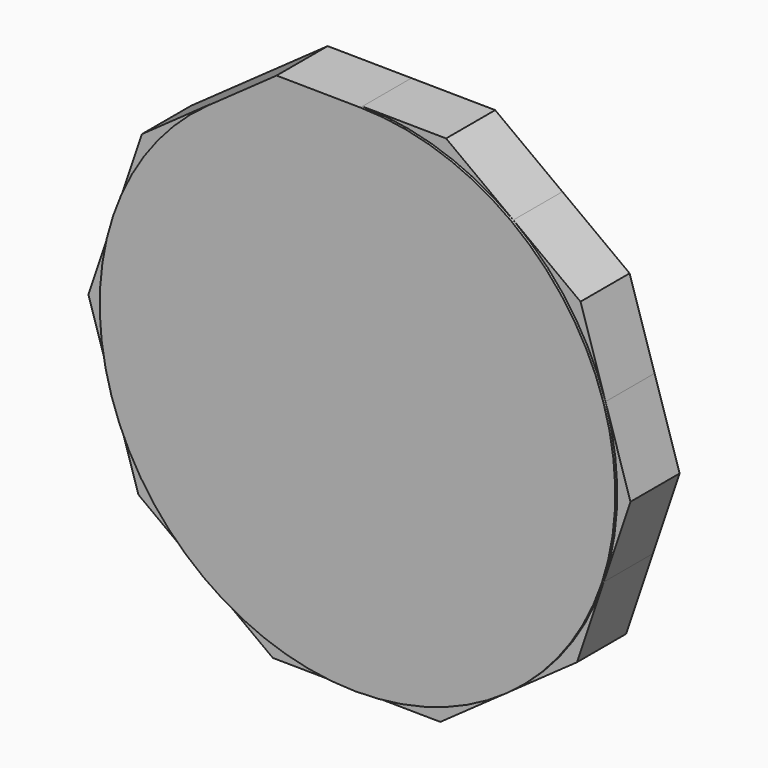
from build123d import *

# Parameters (mm, degrees)
F1_DEPTH = 1
F2_DEPTH = 25


with BuildPart() as f1:
    # F0 (on Front) → F1 (new body)
    with BuildSketch(Plane.XZ):
        with BuildLine():
            ThreePointArc((99.4907408065, -33.5647507629), (103.6135314153, -17.0069429252), (105, 0))
            ThreePointArc((105, 0), (103.7977584549, 15.8437792124), (100.2185649575, 31.3247384325))
            ThreePointArc((100.2185649575, 31.3247384325), (85.6336425012, 60.7608366629), (62.6663022671, 84.2492407097))
            ThreePointArc((62.6663022671, 84.2492407097), (33.5647485771, 99.4907415439), (1.1776435614, 104.9933957716))
            ThreePointArc((1.1776435614, 104.9933957716), (-31.3247392722, 100.218564695), (-60.7608381292, 85.6336414608))
            ThreePointArc((-60.7608381292, 85.6336414608), (-84.2492404255, 62.6663026493), (-99.4907409959, 33.5647502014))
            ThreePointArc((-99.4907409959, 33.5647502014), (-104.9933957718, 1.1776435403), (-100.2185647541, -31.3247390832))
            ThreePointArc((-100.2185647541, -31.3247390832), (-85.6336424849, -60.7608366859), (-62.6663027691, -84.2492403363))
            ThreePointArc((-62.6663027691, -84.2492403363), (-33.5647485613, -99.4907415492), (-1.1776429024, -104.9933957789))
            ThreePointArc((-1.1776429024, -104.9933957789), (31.3247396024, -100.2185645918), (60.7608381561, -85.6336414417))
            ThreePointArc((60.7608381561, -85.6336414417), (84.2492402585, -62.6663028738), (99.4907408065, -33.5647507629))
        make_face()
        with BuildLine():
            ThreePointArc((-60.7608381292, 85.6336414608), (-31.3247392722, 100.218564695), (1.1776435614, 104.9933957716))
            Line((1.1776435614, 104.9933957716), (-32.9367799888, 105.3760349567))
            Line((-32.9367799888, 105.3760349567), (-60.7608381292, 85.6336414608))
        make_face()
    extrude(amount=F1_DEPTH)

    # F0 (on Front) + F1_face (on face) → F2 (join)
    with BuildSketch(Plane.XZ):
        with BuildLine():
            ThreePointArc((99.4907408065, -33.5647507629), (103.6135314153, -17.0069429252), (105, 0))
            ThreePointArc((105, 0), (103.7977584549, 15.8437792124), (100.2185649575, 31.3247384325))
            ThreePointArc((100.2185649575, 31.3247384325), (85.6336425012, 60.7608366629), (62.6663022671, 84.2492407097))
            ThreePointArc((62.6663022671, 84.2492407097), (33.5647485771, 99.4907415439), (1.1776435614, 104.9933957716))
            ThreePointArc((1.1776435614, 104.9933957716), (-31.3247392722, 100.218564695), (-60.7608381292, 85.6336414608))
            ThreePointArc((-60.7608381292, 85.6336414608), (-84.2492404255, 62.6663026493), (-99.4907409959, 33.5647502014))
            ThreePointArc((-99.4907409959, 33.5647502014), (-104.9933957718, 1.1776435403), (-100.2185647541, -31.3247390832))
            ThreePointArc((-100.2185647541, -31.3247390832), (-85.6336424849, -60.7608366859), (-62.6663027691, -84.2492403363))
            ThreePointArc((-62.6663027691, -84.2492403363), (-33.5647485613, -99.4907415492), (-1.1776429024, -104.9933957789))
            ThreePointArc((-1.1776429024, -104.9933957789), (31.3247396024, -100.2185645918), (60.7608381561, -85.6336414417))
            ThreePointArc((60.7608381561, -85.6336414417), (84.2492402585, -62.6663028738), (99.4907408065, -33.5647507629))
        make_face()
        with BuildLine():
            ThreePointArc((100.2185649575, 31.3247384325), (103.7977584549, 15.8437792124), (105, 0))
            ThreePointArc((105, 0), (103.6135314153, -17.0069429252), (99.4907408065, -33.5647507629))
            Line((99.4907408065, -33.5647507629), (110.3965894634, -1.2382463674))
            Line((110.3965894634, -1.2382463674), (100.2185649575, 31.3247384325))
        make_face()
        with BuildLine():
            ThreePointArc((62.6663022671, 84.2492407097), (85.6336425012, 60.7608366629), (100.2185649575, 31.3247384325))
            Line((100.2185649575, 31.3247384325), (90.0405399504, 63.8877248356))
            Line((90.0405399504, 63.8877248356), (62.6663022671, 84.2492407097))
        make_face()
        with BuildLine():
            Line((88.5848940435, -65.8912495444), (99.4907408065, -33.5647507629))
            ThreePointArc((99.4907408065, -33.5647507629), (84.2492402585, -62.6663028738), (60.7608381561, -85.6336414417))
            Line((60.7608381561, -85.6336414417), (88.5848940435, -65.8912495444))
        make_face()
        with BuildLine():
            ThreePointArc((1.1776435614, 104.9933957716), (33.5647485771, 99.4907415439), (62.6663022671, 84.2492407097))
            Line((62.6663022671, 84.2492407097), (35.2920645417, 104.6107566152))
            Line((35.2920645417, 104.6107566152), (1.1776435614, 104.9933957716))
        make_face()
        with BuildLine():
            Line((32.9367799888, -105.3760349567), (60.7608381561, -85.6336414417))
            ThreePointArc((60.7608381561, -85.6336414417), (31.3247396024, -100.2185645918), (-1.1776429024, -104.9933957789))
            Line((-1.1776429024, -104.9933957789), (32.9367799888, -105.3760349567))
        make_face()
        with BuildLine():
            ThreePointArc((-60.7608381292, 85.6336414608), (-31.3247392722, 100.218564695), (1.1776435614, 104.9933957716))
            Line((1.1776435614, 104.9933957716), (-32.9367799888, 105.3760349567))
            Line((-32.9367799888, 105.3760349567), (-60.7608381292, 85.6336414608))
        make_face()
        with BuildLine():
            Line((-35.2920645417, -104.6107566152), (-1.1776429024, -104.9933957789))
            ThreePointArc((-1.1776429024, -104.9933957789), (-33.5647485613, -99.4907415492), (-62.6663027691, -84.2492403363))
            Line((-62.6663027691, -84.2492403363), (-35.2920645417, -104.6107566152))
        make_face()
        with BuildLine():
            ThreePointArc((-99.4907409959, 33.5647502014), (-84.2492404255, 62.6663026493), (-60.7608381292, 85.6336414608))
            Line((-60.7608381292, 85.6336414608), (-88.5848940435, 65.8912495444))
            Line((-88.5848940435, 65.8912495444), (-99.4907409959, 33.5647502014))
        make_face()
        with BuildLine():
            Line((-90.0405399504, -63.8877248356), (-62.6663027691, -84.2492403363))
            ThreePointArc((-62.6663027691, -84.2492403363), (-85.6336424849, -60.7608366859), (-100.2185647541, -31.3247390832))
            Line((-100.2185647541, -31.3247390832), (-90.0405399504, -63.8877248356))
        make_face()
        with BuildLine():
            ThreePointArc((-100.2185647541, -31.3247390832), (-104.9933957718, 1.1776435403), (-99.4907409959, 33.5647502014))
            Line((-99.4907409959, 33.5647502014), (-110.3965894634, 1.2382463674))
            Line((-110.3965894634, 1.2382463674), (-100.2185647541, -31.3247390832))
        make_face()
    with BuildSketch(Plane(origin=(-0.1080602071, -1, 0.3457215964), x_dir=(1, 0, 0), z_dir=(0, -1, 0))):
        with BuildLine():
            Line((1.2857037684, 104.6476741752), (-32.8287197817, 105.0303133603))
            Line((-32.8287197817, 105.0303133603), (-60.6527779221, 85.2879198644))
            ThreePointArc((-60.6527779221, 85.2879198644), (31.4327994792, -100.5642862914), (1.2857037684, 104.6476741752))
        make_face()
    extrude(amount=F2_DEPTH)


solid = f1.part
